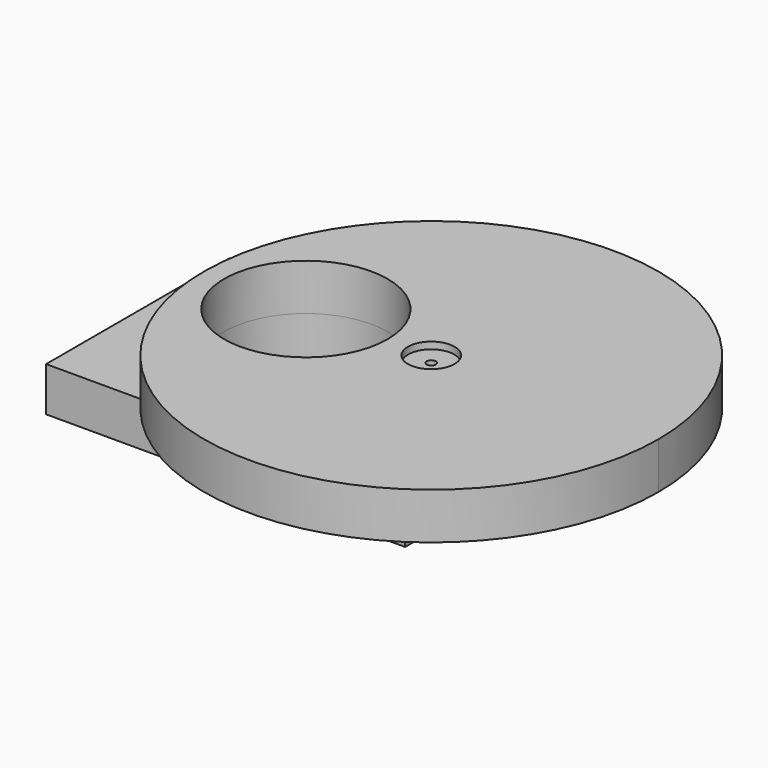
from build123d import *

# Parameters (mm, degrees)
F0_R     = 46.9107423569
F0_R_2   = 13.401249698
F1_DEPTH = 26.67
F0_R_3   = 13.1750226466
F0_R_4   = 6.6660151199
F2_DEPTH = 25.4
F0_R_5   = 2.5920243027
F3_DEPTH = 22.86


with BuildPart() as f1:
    # F0 (on Top) → F1 (new body)
    with BuildSketch(Plane.XY):
        with BuildLine():
            ThreePointArc((180.9600731002, 0), (79.8387593607, 127.0743864177), (-66.6978861635, 57.0713058114))
            Line((-66.6978861635, 57.0713058114), (95.1269119978, 57.0713058114))
            Line((95.1269119978, 57.0713058114), (95.1269119978, -74.433542788))
            Line((95.1269119978, -74.433542788), (-56.5198592453, -74.433542788))
            ThreePointArc((-56.5198592453, -74.433542788), (89.5572424471, -124.4357972599), (180.9600731002, 0))
        make_face()
        with BuildLine():
            Line((95.1269119978, 57.0713058114), (-66.6978861635, 57.0713058114))
            ThreePointArc((-66.6978861635, 57.0713058114), (-79.4607979805, -10.0627966389), (-56.5198592453, -74.433542788))
            Line((-56.5198592453, -74.433542788), (95.1269119978, -74.433542788))
            Line((95.1269119978, -74.433542788), (95.1269119978, 57.0713058114))
        make_face()
        with Locations((-21.4103162289, 0)):
            Circle(F0_R, mode=Mode.SUBTRACT)
        with Locations((50.5552217364, 0)):
            Circle(F0_R_2, mode=Mode.SUBTRACT)
    extrude(amount=F1_DEPTH)


with BuildPart() as f2:
    # F0 (on Top) → F2 (new body)
    with BuildSketch(Plane.XY):
        with BuildLine():
            Line((-66.6978861635, 57.0713058114), (-110.9738275409, 57.0713058114))
            Line((-110.9738275409, 57.0713058114), (-110.9738275409, -74.433542788))
            Line((-110.9738275409, -74.433542788), (-56.5198592453, -74.433542788))
            ThreePointArc((-56.5198592453, -74.433542788), (-79.4607979805, -10.0627966389), (-66.6978861635, 57.0713058114))
        make_face()
        with BuildLine():
            Line((95.1269119978, 57.0713058114), (-66.6978861635, 57.0713058114))
            ThreePointArc((-66.6978861635, 57.0713058114), (-79.4607979805, -10.0627966389), (-56.5198592453, -74.433542788))
            Line((-56.5198592453, -74.433542788), (95.1269119978, -74.433542788))
            Line((95.1269119978, -74.433542788), (95.1269119978, 57.0713058114))
        make_face()
        with Locations((-21.4103162289, 0)):
            Circle(F0_R, mode=Mode.SUBTRACT)
        with Locations((50.5552217364, 0)):
            Circle(F0_R_2, mode=Mode.SUBTRACT)
        with Locations((50.5552217364, 0)):
            Circle(F0_R_2)
        with Locations((50.5552217364, 0)):
            Circle(F0_R_3, mode=Mode.SUBTRACT)
        with Locations((50.5552217364, 0)):
            Circle(F0_R_3)
        with Locations((50.5552217364, 0)):
            Circle(F0_R_4, mode=Mode.SUBTRACT)
    extrude(amount=-F2_DEPTH)

    # F0 (on Top) → F3 (join)
    with BuildSketch(Plane.XY):
        with Locations((50.5552217364, 0)):
            Circle(F0_R_3)
        with Locations((50.5552217364, 0)):
            Circle(F0_R_4, mode=Mode.SUBTRACT)
        with Locations((50.5552217364, 0)):
            Circle(F0_R_4)
        with Locations((50.5552217364, 0)):
            Circle(F0_R_5, mode=Mode.SUBTRACT)
    extrude(amount=F3_DEPTH)


solid = Compound([f1.part, f2.part])
